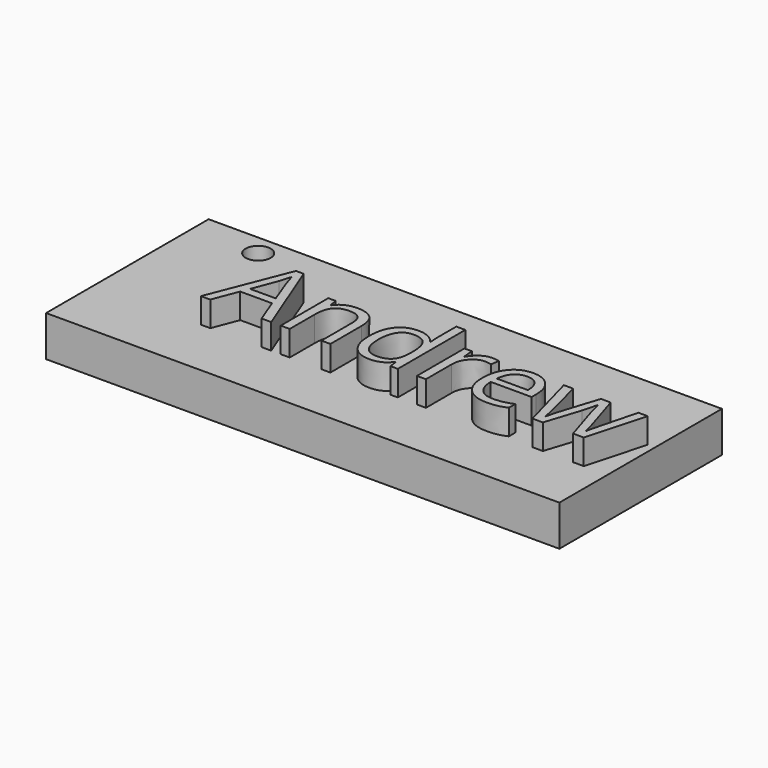
from build123d import *

# Parameters (mm, degrees)
F0_W         = 320.8197380684
F0_H         = 127
F2_DEPTH     = 25.4
F1_TEXT_SIZE = 69.3870582209
F3_DEPTH     = 41.148
F4_R         = 7.8385802127
F5_DEPTH     = 156.718


# Not quite as in the source:
# - Text() gives the source's letters only with a copy of the font that has no kerning and outlines rounded to 1/6400 em; it was checked with that copy


with BuildPart() as f2:
    # F0 (on Top) → F2 (new body)
    with BuildSketch(Plane.XY):
        with Locations((-26.7249718308, 12.8393443301)):
            Rectangle(F0_W, F0_H)
    extrude(amount=F2_DEPTH)

    # F1 (on face) → F3 (join)
    with BuildSketch(Plane.XY):
        with Locations((-120.3789115479, -13.1034673048)):
            Text('Andrew', F1_TEXT_SIZE, font='Open Sans', text_align=(TextAlign.LEFT, TextAlign.BOTTOM))
    extrude(amount=F3_DEPTH)

    # F4 (on face) → F5 (cut)
    with BuildSketch(Plane.XY.offset(25.4)):
        with Locations((-145.7779556513, 63.3594170213)):
            Circle(F4_R)
    extrude(amount=-F5_DEPTH, mode=Mode.SUBTRACT)


solid = f2.part
